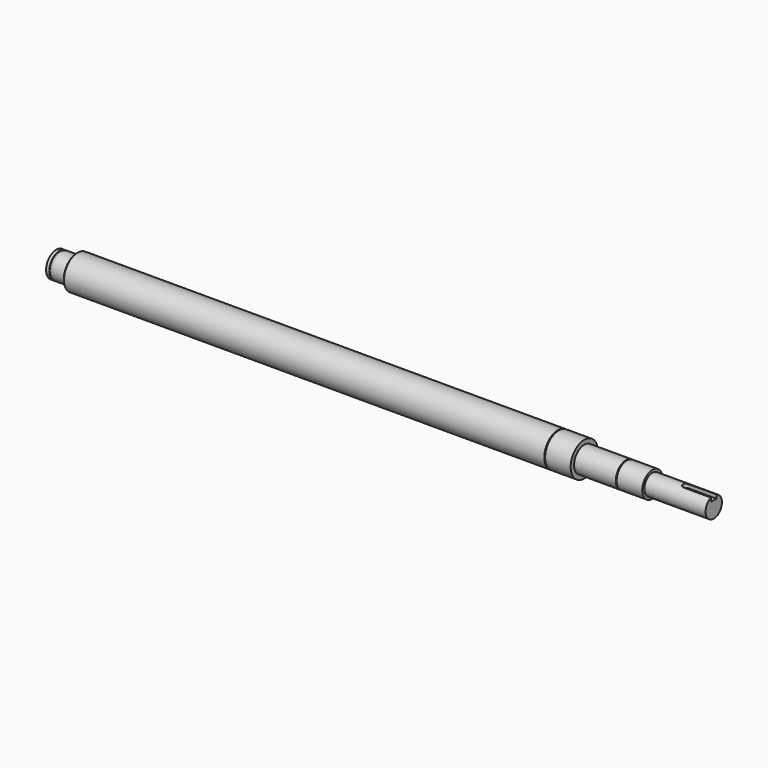
from build123d import *

# Parameters (mm, degrees)
F0_R      = 7.5
F1_DEPTH  = 9
F2_R      = 7.15
F3_DEPTH  = 1.15
F4_R      = 7.5
F5_DEPTH  = 1.85
F6_R      = 10
F7_DEPTH  = 283
F8_SIZE   = 0.5
F9_R      = 10
F10_DEPTH = 15
F11_R     = 7.5
F12_DEPTH = 25
F13_SIZE  = 0.5
F14_R     = 7.5
F15_DEPTH = 15
F16_R     = 6
F17_DEPTH = 36
F19_W     = 18
F19_H     = 4
F20_DEPTH = 2.5
F21_R     = 1.9999


# Not quite as in the source:
# - a fillet or chamfer is up to 0.001 mm smaller than in the source, because OpenCascade refuses the exact size


with BuildPart() as f1:
    # F0 (on Right) → F1 (new body)
    with BuildSketch(Plane.YZ):
        Circle(F0_R)
    extrude(amount=-F1_DEPTH)

    # F2 (on face) → F3 (join)
    with BuildSketch(Plane(origin=(-9, 0, 0), x_dir=(0, -1, 0), z_dir=(-1, 0, 0))):
        Circle(F2_R)
    extrude(amount=F3_DEPTH)

    # F4 (on face) → F5 (join)
    with BuildSketch(Plane(origin=(-10.15, 0, 0), x_dir=(0, -1, 0), z_dir=(-1, 0, 0))):
        Circle(F4_R)
    extrude(amount=F5_DEPTH)

    # F6 (on Right) → F7 (join)
    with BuildSketch(Plane.YZ):
        Circle(F6_R)
    extrude(amount=F7_DEPTH)

    # F8
    f8_edges = [f1.edges().sort_by_distance(p)[0] for p in [
        (283, -10, 0),
        (0, -10, 0),
    ]]
    chamfer(f8_edges, length=F8_SIZE)

    # F9 (on face) → F10 (join)
    with BuildSketch(Plane.YZ.offset(283)):
        Circle(F9_R)
    extrude(amount=F10_DEPTH)

    # F11 (on face) → F12 (join)
    with BuildSketch(Plane.YZ.offset(298)):
        Circle(F11_R)
    extrude(amount=F12_DEPTH)

    # F13
    f13_edges = [f1.edges().sort_by_distance(p)[0] for p in [
        (323, -7.5, 0),
    ]]
    chamfer(f13_edges, length=F13_SIZE)

    # F14 (on face) → F15 (join)
    with BuildSketch(Plane.YZ.offset(323)):
        Circle(F14_R)
    extrude(amount=F15_DEPTH)

    # F16 (on face) → F17 (join)
    with BuildSketch(Plane.YZ.offset(338)):
        Circle(F16_R)
    extrude(amount=F17_DEPTH)

    # F19 (on offset) → F20 (cut)
    with BuildSketch(Plane.XY.offset(6)):
        with Locations((365, 0)):
            Rectangle(F19_W, F19_H)
    extrude(amount=-F20_DEPTH, mode=Mode.SUBTRACT)

    # F21 (radius 2 in the source; OpenCascade refuses exactly that, so slightly less here)
    f21_edges = [f1.edges().sort_by_distance(p)[0] for p in [
        (356, 2, 4.578427),
        (356, -2, 4.578427),
    ]]
    fillet(f21_edges, radius=F21_R)


solid = f1.part
